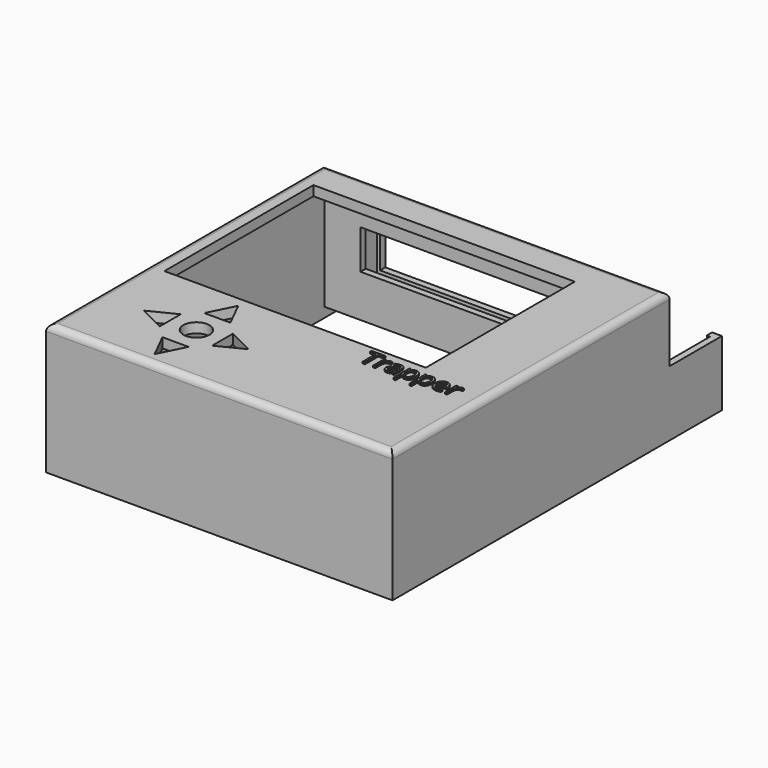
from build123d import *

# Parameters (mm, degrees)
F0_W           = 106
F0_H           = 106
F1_DEPTH       = 40
F2_W           = 102
F2_H           = 102
F3_DEPTH       = 37
F4_W           = 80
F4_H           = 57
F4_R           = 4
F5_DEPTH       = 3
F6_R           = 2
F7_TEXT_SIZE   = 7.9717666597
F8_DEPTH       = 0.5
F9_W           = 20.0079137683
F9_H           = 20
F10_DEPTH      = 106
F11_W          = 102
F11_H          = 16
F12_DEPTH      = 25
F12_DEPTH_BACK = 25
F13_W          = 100
F13_H          = 15
F14_DEPTH      = 20
F15_W          = 102
F15_H          = 4
F15_H_2        = 16
F16_DEPTH      = 3
F17_W          = 80
F17_H          = 12
F18_DEPTH      = 5


# Not quite as in the source:
# - Text() gives the source's letters only with a copy of the font that has no kerning and outlines rounded to 1/6400 em; it was checked with that copy


with BuildPart() as f1:
    # F0 (on Top) → F1 (new body)
    with BuildSketch(Plane.XY):
        with Locations((53, 53)):
            Rectangle(F0_W, F0_H)
    extrude(amount=F1_DEPTH)

    # F2 (on face) → F3 (cut)
    with BuildSketch(Plane(origin=(0, 0, 0), x_dir=(1, 0, 0), z_dir=(0, 0, -1))):
        with Locations((53, -53)):
            Rectangle(F2_W, F2_H)
    extrude(amount=-F3_DEPTH, mode=Mode.SUBTRACT)

    # F4 (on face) → F5 (cut, through all)
    with BuildSketch(Plane.XY.offset(40)):
        with Locations((45, 67.5)):
            Rectangle(F4_W, F4_H)
        with Locations((30, 20)):
            Circle(F4_R)
        Polygon((46, 20), (38, 24), (38, 16), align=None)
        Polygon((30, 36), (26, 28), (34, 28), align=None)
        Polygon((14, 20), (22, 16), (22, 24), align=None)
        Polygon((34, 12), (26, 12), (30, 4), align=None)
    extrude(amount=-F5_DEPTH, mode=Mode.SUBTRACT)

    # F6
    f6_edges = [f1.edges().sort_by_distance(p)[0] for p in [
        (53, 106, 40),
        (0, 53, 40),
        (53, 0, 40),
        (106, 53, 40),
    ]]
    fillet(f6_edges, radius=F6_R)

    # F7 (on face) → F8 (join)
    with BuildSketch(Plane.XY.offset(40)):
        with Locations((70, 31.260328005)):
            Text('Trapper', F7_TEXT_SIZE, font='Open Sans', text_align=(TextAlign.LEFT, TextAlign.BOTTOM))
    extrude(amount=F8_DEPTH)

    # F9 (on Right) → F10 (join)
    with BuildSketch(Plane.YZ):
        with Locations((115.9960431159, 10)):
            Rectangle(F9_W, F9_H)
    extrude(amount=F10_DEPTH)

    # F11 (on Top) → F12 (cut, two sides)
    with BuildSketch(Plane.XY) as f12_sk:
        with Locations((53, 116)):
            Rectangle(F11_W, F11_H)
    extrude(amount=-F12_DEPTH, mode=Mode.SUBTRACT)
    extrude(f12_sk.sketch, amount=F12_DEPTH_BACK, mode=Mode.SUBTRACT)

    # F13 (on face) → F14 (cut)
    with BuildSketch(Plane(origin=(0, 126, 0), x_dir=(-1, 0, 0), z_dir=(0, 1, 0))):
        with Locations((-53, 12.5)):
            Rectangle(F13_W, F13_H)
    extrude(amount=-F14_DEPTH, mode=Mode.SUBTRACT)

    # F15 (on face) → F16 (cut)
    with BuildSketch(Plane(origin=(0, 0, 0), x_dir=(1, 0, 0), z_dir=(0, 0, -1))):
        with Locations((53, -106)):
            Rectangle(F15_W, F15_H)
        with Locations((53, -116)):
            Rectangle(F15_W, F15_H_2)
    extrude(amount=-F16_DEPTH, mode=Mode.SUBTRACT)

    # F17 (on face) → F18 (cut)
    with BuildSketch(Plane(origin=(0, 106, 0), x_dir=(-1, 0, 0), z_dir=(0, 1, 0))):
        with Locations((-53, 22)):
            Rectangle(F17_W, F17_H)
    extrude(amount=-F18_DEPTH, mode=Mode.SUBTRACT)


solid = f1.part
